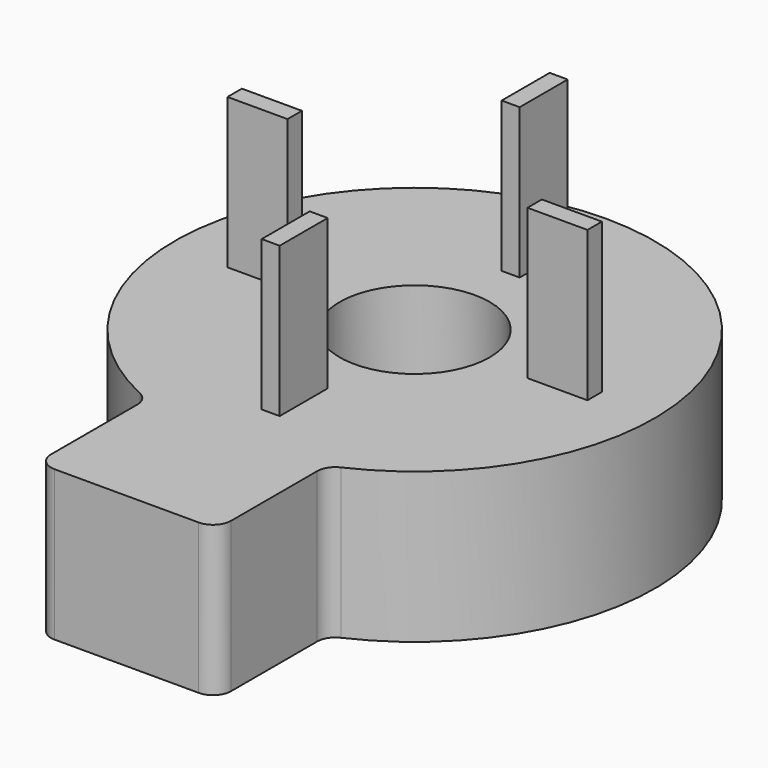
from build123d import *

# Parameters (mm, degrees)
F1_DEPTH        = 25
F2_R            = 12.5
F3_DEPTH        = 15
F4_W            = 10
F4_H            = 25
F5_DEPTH        = 1.5
F5_COPIES_COUNT = 4


# Not quite as in the source:
# - a pattern or mirror of a feature is missing from the dataset's text; its kind, count and spacing are read off the source's solid


with BuildPart() as f1:
    # F0 (on Top) → F1 (new body)
    with BuildSketch(Plane.XY):
        with BuildLine():
            ThreePointArc((15, -39.0512483795), (15.4733973541, -37.4337567815), (16.7441860465, -36.3267426786))
            ThreePointArc((16.7441860465, -36.3267426786), (0, 40), (-16.7441860465, -36.3267426786))
            ThreePointArc((-16.7441860465, -36.3267426786), (-15.4733973541, -37.4337567815), (-15, -39.0512483795))
            Line((-15, -39.0512483795), (-15, -57))
            ThreePointArc((-15, -57), (-14.1213203436, -59.1213203436), (-12, -60))
            Line((-12, -60), (12, -60))
            ThreePointArc((12, -60), (14.1213203436, -59.1213203436), (15, -57))
            Line((15, -57), (15, -39.0512483795))
        make_face()
    extrude(amount=F1_DEPTH)

    # F2 (on face) → F3 (cut)
    with BuildSketch(Plane.XY.offset(25)):
        Circle(F2_R)
    extrude(amount=-F3_DEPTH, mode=Mode.SUBTRACT)

    # F4 (on Right) → F5 (join, symmetric)
    with BuildSketch(Plane.YZ):
        with Locations((-25, 37.5)):
            Rectangle(F4_W, F4_H)
    f5 = extrude(amount=F5_DEPTH, both=True)

    # F5_copies: F5 ×4 about axis
    f5_copies_axis = Axis((0, 0, 0), (0, 0, 1))
    for i in range(1, F5_COPIES_COUNT):
        add(f5.rotate(f5_copies_axis, i * 360 / F5_COPIES_COUNT))


solid = f1.part
